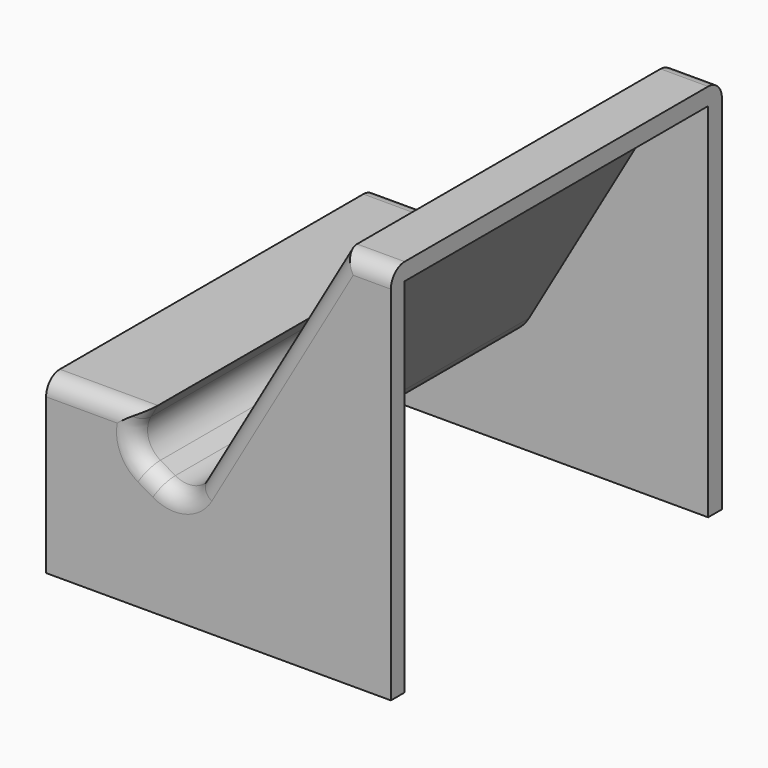
from build123d import *

# Parameters (mm, degrees)
F0_W         = 60
F0_H         = 30
F1_DEPTH     = 60
F2_R         = 7.5
F3_T1_DEPTH  = 38.8119784648
F3_T3_DEPTH  = 97.3760430703
F3_T5_DEPTH  = 5
F3_T7_DEPTH  = 16.5470053838
F3_T9_DEPTH  = 53.4529946162
F3_T12_ANGLE = 90
F3_T14_ANGLE = 90
F3_T16_ANGLE = 90
F3_T18_ANGLE = 90
F4_T         = 5


# Not quite as in the source:
# - a fillet or chamfer that OpenCascade refuses, or shapes differently, is made with other operations: its cross-section is extruded or revolved along the edge and cut away or added
# - a shell that OpenCascade refuses in one call is made with other operations: the cavity is built on its own and cut out


with BuildPart() as f1:
    # F0 (on Front) → F1 (new body, symmetric)
    with BuildSketch(Plane.XZ):
        Polygon((46.1880215352, 80), (0, 0), (60, 0), (60, 80), align=None)
        with Locations((30, -15)):
            Rectangle(F0_W, F0_H)
        Polygon((0, -30), (0, 0), (-17.3205080757, 10), (-11.5470053838, 20), (-40, 20), (-40, -30), align=None)
    extrude(amount=F1_DEPTH, both=True)

    # F2
    f2_edges = [f1.edges().sort_by_distance(p)[0] for p in [
        (-17.320508, 0, 10),
        (0, 0, 0),
    ]]
    fillet(f2_edges, radius=F2_R)

    # F3: fillet of radius 5 on 14 edges, made by hand

    # F3_s2 → F3_t1 (cut)
    with BuildSketch(Plane.YZ.offset(33.6880215352)):
        with BuildLine():
            ThreePointArc((-55, 80), (-58.5355339059, 78.5355339059), (-60, 75))
            Line((-60, 75), (-60, 80))
            Line((-60, 80), (-55, 80))
        make_face()
        with BuildLine():
            ThreePointArc((60, 75), (58.5355339059, 78.5355339059), (55, 80))
            Line((55, 80), (60, 80))
            Line((60, 80), (60, 75))
        make_face()
    extrude(amount=F3_T1_DEPTH, mode=Mode.SUBTRACT)

    # F3_s4 → F3_t3 (cut)
    with BuildSketch(Plane(origin=(52.4380215352, 0, 90.8253175473), x_dir=(0, 1, 0), z_dir=(-0.5, 0, -0.8660254038))):
        with BuildLine():
            ThreePointArc((-55, 0), (-58.5355339059, 1.4644660941), (-60, 5))
            Line((-60, 5), (-60, 0))
            Line((-60, 0), (-55, 0))
        make_face()
        with BuildLine():
            ThreePointArc((55, 0), (58.5355339059, 1.4644660941), (60, 5))
            Line((60, 5), (60, 0))
            Line((60, 0), (55, 0))
        make_face()
    extrude(amount=F3_T3_DEPTH, mode=Mode.SUBTRACT)

    # F3_s6 → F3_t5 (cut)
    with BuildSketch(Plane(origin=(-6.4951905284, 0, 3.75), x_dir=(0, 1, 0), z_dir=(-0.8660254038, 0, 0.5))):
        with BuildLine():
            ThreePointArc((-60, 5), (-58.5355339059, 1.4644660941), (-55, 0))
            Line((-55, 0), (-60, 0))
            Line((-60, 0), (-60, 5))
        make_face()
        with BuildLine():
            ThreePointArc((60, 5), (58.5355339059, 1.4644660941), (55, 0))
            Line((55, 0), (60, 0))
            Line((60, 0), (60, 5))
        make_face()
    extrude(amount=F3_T5_DEPTH, mode=Mode.SUBTRACT)

    # F3_s8 → F3_t7 (cut)
    with BuildSketch(Plane(origin=(3.75, 0, 6.4951905284), x_dir=(0, 1, 0), z_dir=(0.5, 0, 0.8660254038))):
        with BuildLine():
            ThreePointArc((-60, 25), (-58.5355339059, 21.4644660941), (-55, 20))
            Line((-55, 20), (-60, 20))
            Line((-60, 20), (-60, 25))
        make_face()
        with BuildLine():
            ThreePointArc((60, 25), (58.5355339059, 21.4644660941), (55, 20))
            Line((55, 20), (60, 20))
            Line((60, 20), (60, 25))
        make_face()
    extrude(amount=F3_T7_DEPTH, mode=Mode.SUBTRACT)

    # F3_s10 → F3_t9 (cut)
    with BuildSketch(Plane.YZ.offset(-52.5)):
        with BuildLine():
            ThreePointArc((-60, 15), (-58.5355339059, 18.5355339059), (-55, 20))
            Line((-55, 20), (-60, 20))
            Line((-60, 20), (-60, 15))
        make_face()
        with BuildLine():
            ThreePointArc((60, 15), (58.5355339059, 18.5355339059), (55, 20))
            Line((55, 20), (60, 20))
            Line((60, 20), (60, 15))
        make_face()
    extrude(amount=F3_T9_DEPTH, mode=Mode.SUBTRACT)

    # F3_s11 → F3_t12 (revolve, cut)
    with BuildSketch(Plane(origin=(3.75, 0, 6.4951905284), x_dir=(0, 1, 0), z_dir=(0.5, 0, 0.8660254038))):
        with BuildLine():
            ThreePointArc((60, -5), (58.5355339059, -1.4644660941), (55, 0))
            Line((55, 0), (60, 0))
            Line((60, 0), (60, -5))
        make_face()
    revolve(axis=Axis((-2.7451905284, 60, 10.2451905284), (0, 1, 0)), revolution_arc=F3_T12_ANGLE, mode=Mode.SUBTRACT)

    # F3_s13 → F3_t14 (revolve, cut)
    with BuildSketch(Plane(origin=(3.75, 0, 6.4951905284), x_dir=(0, 1, 0), z_dir=(0.5, 0, 0.8660254038))):
        with BuildLine():
            ThreePointArc((60, 25), (58.5355339059, 21.4644660941), (55, 20))
            Line((55, 20), (60, 20))
            Line((60, 20), (60, 25))
        make_face()
    revolve(axis=Axis((-7.0753175473, 60, 12.7451905284), (0, -1, 0)), revolution_arc=F3_T14_ANGLE, mode=Mode.SUBTRACT)

    # F3_s15 → F3_t16 (revolve, cut)
    with BuildSketch(Plane(origin=(3.75, 0, 6.4951905284), x_dir=(0, 1, 0), z_dir=(0.5, 0, 0.8660254038))):
        with BuildLine():
            ThreePointArc((-55, 0), (-58.5355339059, -1.4644660941), (-60, -5))
            Line((-60, -5), (-60, 0))
            Line((-60, 0), (-55, 0))
        make_face()
    revolve(axis=Axis((-2.7451905284, -60, 10.2451905284), (0, 1, 0)), revolution_arc=F3_T16_ANGLE, mode=Mode.SUBTRACT)

    # F3_s17 → F3_t18 (revolve, cut)
    with BuildSketch(Plane(origin=(3.75, 0, 6.4951905284), x_dir=(0, 1, 0), z_dir=(0.5, 0, 0.8660254038))):
        with BuildLine():
            ThreePointArc((-60, 25), (-58.5355339059, 21.4644660941), (-55, 20))
            Line((-55, 20), (-60, 20))
            Line((-60, 20), (-60, 25))
        make_face()
    revolve(axis=Axis((-7.0753175473, -60, 12.7451905284), (0, -1, 0)), revolution_arc=F3_T18_ANGLE, mode=Mode.SUBTRACT)

    # F4: shell of thickness 5, made by hand


with BuildPart() as f4_core1:
    # F4_t2: copy of F1
    add(f1.part)

    # the walls: a layer under each face that stays
    f4_faces = [f4_core1.faces().sort_by_distance(p)[0] for p in [
        (24.9690107676, 0, 43.2475952642),
        (53.0940107676, 0, 80),
        (-0.8040476901, 0, 3.0007468312),
        (-23.3333333333, -60, -12.5),
        (-8.6602540378, 0, 5),
        (-23.3333333333, 60, -12.5),
        (-14.3197612445, 0, 10.8040476901),
        (-25.7735026919, 0, 20),
        (-12.5587567297, 0, 18.2475952642),
    ]]
    thicken(f4_faces, amount=-F4_T, mode=Mode.SUBTRACT)


with BuildPart() as f1_1:
    add(f1.part)

    # what is left inside the walls is the cavity
    f4_cavity = [f4_core1.part.solids().sort_by_distance(p)[0] for p in [
        (59.95, 18.333333, 22.5),
    ]]
    add(f4_cavity, mode=Mode.SUBTRACT)


solid = f1_1.part
